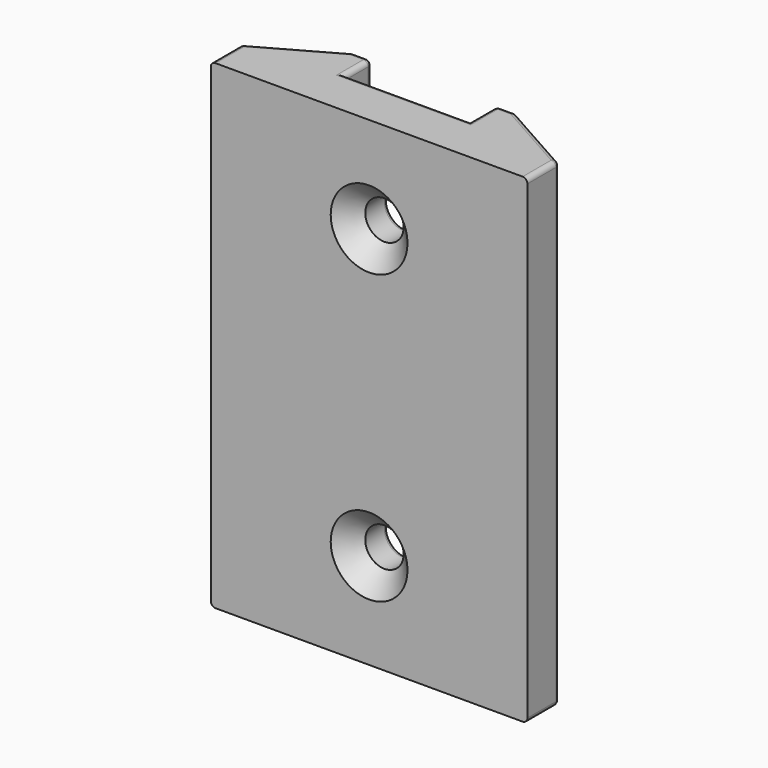
from build123d import *

# Parameters (mm, degrees)
F0_W           = 12
F0_H           = 50
F0_R           = 2
F0_W_2         = 0.5
F0_W_3         = 10
F1_DEPTH       = 5
F2_DEPTH       = 8.5
F3_SIZE2       = 8
F3_SIZE        = 4.5
F4_SIZE2       = 8
F4_SIZE        = 4.5
F5_D           = 4
F5_CSINK_D     = 8
F5_CSINK_ANGLE = 90
F6_R           = 0.5


with BuildPart() as f1:
    # F0 (on Front) → F1 (new body)
    with BuildSketch(Plane.XZ):
        Rectangle(F0_W, F0_H)
        with Locations((0, -15)):
            Circle(F0_R, mode=Mode.SUBTRACT)
        with Locations((0, 15)):
            Circle(F0_R, mode=Mode.SUBTRACT)
        with Locations((6.25, 0)):
            Rectangle(F0_W_2, F0_H)
        with Locations((-6.25, 0)):
            Rectangle(F0_W_2, F0_H)
        with Locations((11.5, 0)):
            Rectangle(F0_W_3, F0_H)
        with Locations((-11.5, 0)):
            Rectangle(F0_W_3, F0_H)
    extrude(amount=-F1_DEPTH)

    # F0 (on Front) → F2 (join)
    with BuildSketch(Plane.XZ):
        with Locations((-11.5, 0)):
            Rectangle(F0_W_3, F0_H)
        with Locations((11.5, 0)):
            Rectangle(F0_W_3, F0_H)
    extrude(amount=-F2_DEPTH)

    # F3
    f3_edges = [f1.edges().sort_by_distance(p)[0] for p in [
        (-16.5, 8.5, 0),
    ]]
    f3_side = f1.faces().sort_by_distance((-16.5, 4.25, 0))[0]
    chamfer(f3_edges, length=F3_SIZE, length2=F3_SIZE2, reference=f3_side)

    # F4
    f4_edges = [f1.edges().sort_by_distance(p)[0] for p in [
        (16.5, 8.5, 0),
    ]]
    f4_side = f1.faces().sort_by_distance((16.5, 4.25, 0))[0]
    chamfer(f4_edges, length=F4_SIZE, length2=F4_SIZE2, reference=f4_side)

    # F5 (through all)
    with Locations(Plane.XZ):
        with Locations((0, 15), (0, -15)):
            CounterSinkHole(F5_D / 2, F5_CSINK_D / 2, counter_sink_angle=F5_CSINK_ANGLE)

    # F6
    f6_edges = [f1.edges().sort_by_distance(p)[0] for p in [
        (12.5, 6.25, -25),
        (16.5, 4, 0),
        (8.5, 8.5, 0),
        (12.5, 6.25, 25),
        (7.5, 8.5, -25),
        (6.5, 8.5, 0),
        (7.5, 8.5, 25),
        (-7.5, 8.5, -25),
        (-8.5, 8.5, 0),
        (-6.5, 8.5, 0),
        (-7.5, 8.5, 25),
        (-12.5, 6.25, 25),
        (-16.5, 4, 0),
        (-12.5, 6.25, -25),
        (-2, 5, -15),
        (-2, 5, 15),
        (0, 5, -25),
        (6.5, 6.75, -25),
        (-6.5, 6.75, -25),
        (-16.5, 2, -25),
        (16.5, 2, -25),
        (16.5, 2, 25),
        (6.5, 6.75, 25),
        (0, 5, 25),
        (-6.5, 6.75, 25),
        (-16.5, 2, 25),
    ]]
    fillet(f6_edges, radius=F6_R)


solid = f1.part
